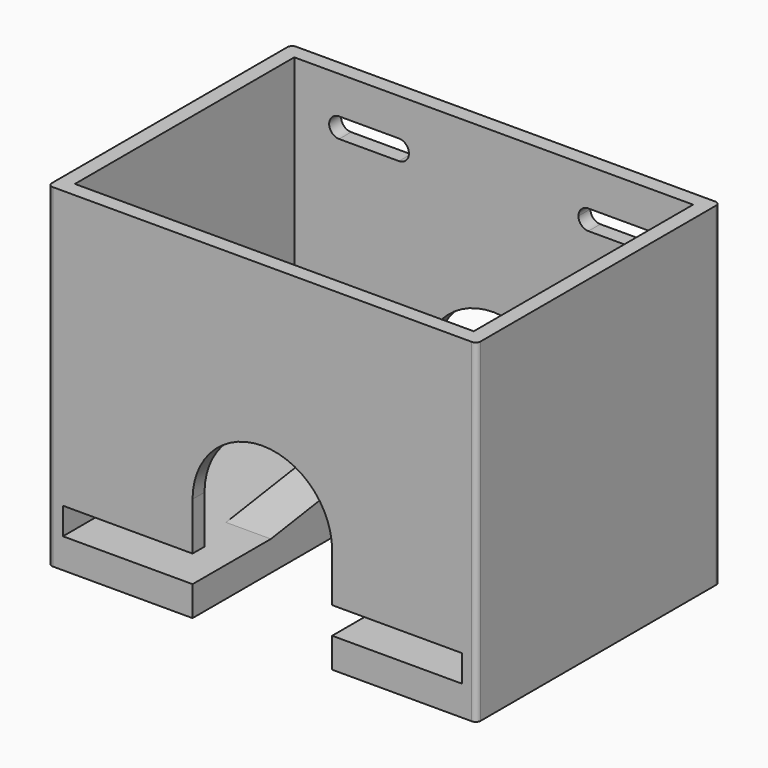
from build123d import *

# Parameters (mm, degrees)
F0_W      = 86
F0_H      = 61
F0_W_2    = 80
F0_H_2    = 55
F1_DEPTH  = 67
F2_DEPTH  = 6
F3_W      = 80
F3_H      = 5.4
F4_DEPTH  = 3
F6_W      = 28
F6_H      = 3
F6_H_2    = 55
F7_DEPTH  = 35
F8_R      = 13.99999
F9_DEPTH  = 23
F10_W     = 28
F10_H     = 29.4785189629
F11_DEPTH = 25
F12_W     = 6
F12_H     = 2
F13_DEPTH = 6
F14_R     = 1


# Not quite as in the source:
# - a fillet or chamfer is up to 0.001 mm smaller than in the source, because OpenCascade refuses the exact size


with BuildPart() as f1:
    # F0 (on Top) → F1 (new body)
    with BuildSketch(Plane.XY):
        Rectangle(F0_W, F0_H)
        Rectangle(F0_W_2, F0_H_2, mode=Mode.SUBTRACT)
    extrude(amount=F1_DEPTH)

    # F0 (on Top) → F2 (join)
    with BuildSketch(Plane.XY):
        Rectangle(F0_W_2, F0_H_2)
    extrude(amount=F2_DEPTH)

    # F3 (on face) → F4 (cut)
    with BuildSketch(Plane.XZ.offset(30.5)):
        with Locations((0, 8.7)):
            Rectangle(F3_W, F3_H)
    extrude(amount=-F4_DEPTH, mode=Mode.SUBTRACT)

    # F6 (on face) → F7 (cut)
    with BuildSketch(Plane.XY):
        with Locations((0, -29)):
            Rectangle(F6_W, F6_H)
        Rectangle(F6_W, F6_H_2)
        with Locations((0, 29)):
            Rectangle(F6_W, F6_H)
    extrude(amount=F7_DEPTH, mode=Mode.SUBTRACT)

    # F8 (radius 14 in the source; OpenCascade refuses exactly that, so slightly less here)
    f8_edges = [f1.edges().sort_by_distance(p)[0] for p in [
        (14, -29, 35),
        (-14, -29, 35),
        (-14, 29, 35),
        (14, 29, 35),
    ]]
    fillet(f8_edges, radius=F8_R)

    # F5 (on Right) → F9 (join, symmetric)
    with BuildSketch(Plane.YZ):
        Polygon((-10.8611155301, 0), (29.1388844699, 0), (29.1388844699, 12), (-10.8611155301, 6), align=None)
    extrude(amount=F9_DEPTH, both=True)

    # F10 (on face) → F11 (cut)
    with BuildSketch(Plane(origin=(0, -1.1191932513, 7.4612883418), x_dir=(1, 0, 0), z_dir=(0, -0.1483404529, 0.9889363529))):
        Polygon((-14, -9.8509092629), (14, -9.8509092629), (14, 28.9393682094), (14, 30.5965875694), (-14, 30.5965875694), (-14, 28.9393682094), align=None)
        with Locations((0, -24.5901687443)):
            Rectangle(F10_W, F10_H)
    extrude(amount=-F11_DEPTH, mode=Mode.SUBTRACT)

    # F12 (on face) → F13 (cut)
    with BuildSketch(Plane(origin=(0, 30.5, 0), x_dir=(-1, 0, 0), z_dir=(0, 1, 0))):
        with BuildLine():
            Line((-31, 55.5), (-31, 59.5))
            ThreePointArc((-31, 59.5), (-33, 57.5), (-31, 55.5))
        make_face()
        Polygon((-25, 57.5), (-19, 57.5), (-19, 59.5), (-31, 59.5), (-31, 55.5), (-25, 55.5), align=None)
        with Locations((-22, 56.5)):
            Rectangle(F12_W, F12_H)
        with BuildLine():
            ThreePointArc((-19, 55.5), (-17.5857864376, 56.0857864376), (-17, 57.5))
            Line((-17, 57.5), (-19, 57.5))
            Line((-19, 57.5), (-19, 55.5))
        make_face()
        with BuildLine():
            Line((-19, 57.5), (-17, 57.5))
            ThreePointArc((-17, 57.5), (-17.5857864376, 58.9142135624), (-19, 59.5))
            Line((-19, 59.5), (-19, 57.5))
        make_face()
        with BuildLine():
            Line((19, 55.5), (19, 57.5))
            Line((19, 57.5), (17, 57.5))
            ThreePointArc((17, 57.5), (17.5857864376, 56.0857864376), (19, 55.5))
        make_face()
        with BuildLine():
            Line((17, 57.5), (19, 57.5))
            Line((19, 57.5), (19, 59.5))
            ThreePointArc((19, 59.5), (17.5857864376, 58.9142135624), (17, 57.5))
        make_face()
        Polygon((19, 57.5), (25, 57.5), (25, 55.5), (31, 55.5), (31, 59.5), (19, 59.5), align=None)
        with Locations((22, 56.5)):
            Rectangle(F12_W, F12_H)
        with BuildLine():
            Line((31, 59.5), (31, 55.5))
            ThreePointArc((31, 55.5), (33, 57.5), (31, 59.5))
        make_face()
    extrude(amount=-F13_DEPTH, mode=Mode.SUBTRACT)

    # F14
    f14_edges = [f1.edges().sort_by_distance(p)[0] for p in [
        (-43, -30.5, 33.5),
        (43, -30.5, 33.5),
        (43, 30.5, 33.5),
        (-43, 30.5, 33.5),
    ]]
    fillet(f14_edges, radius=F14_R)


solid = f1.part
